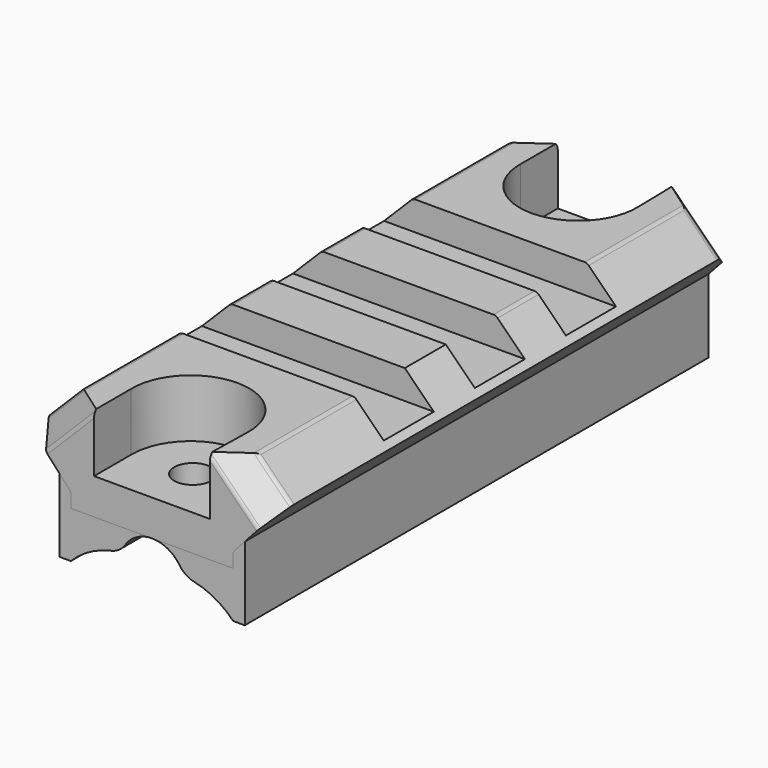
from build123d import *

# Parameters (mm, degrees)
F1_DEPTH  = 25
F2_W      = 28
F2_H      = 5.4
F2_W_2    = 13.9033808853
F2_W_3    = 14.6222274978
F3_DEPTH  = 2.5
F4_SIZE   = 2
F5_R      = 0.5
F8_DEPTH  = 5
F9_R      = 1.6
F10_DEPTH = 3.101
F12_DEPTH = 50
F14_R     = 2
F15_R     = 2
F17_R     = 1.6
F18_DEPTH = 47.90054


# Not quite as in the source:
# - a feature names something its author has since deleted; it is built from what else it names


with BuildPart() as f1:
    # F0 (on Front) → F1 (new body, symmetric)
    with BuildSketch(Plane.XZ):
        Polygon((-7.5, -4.8), (7.5, -4.8), (7.5, -3), (10.5, 0.3), (7.5, 3.3), (-7.5, 3.3), (-10.5, 0.3), (-7.5, -3), align=None)
    extrude(amount=F1_DEPTH, both=True)

    # F2 (on face) → F3 (cut)
    with BuildSketch(Plane.XY.offset(3.3)):
        Rectangle(F2_W, F2_H)
        Polygon((-14.1051735731, 12.5189756917), (-14, 7.12), (14.1193151165, 7.12), (14.1193151165, 12.5189756917), (0, 12.5189756917), align=None)
        with Locations((-6.9516904427, -9.8195246701)):
            Rectangle(F2_W_2, F2_H)
        with Locations((7.3111137489, -9.8195246701)):
            Rectangle(F2_W_3, F2_H)
    extrude(amount=-F3_DEPTH, mode=Mode.SUBTRACT)

    # F4
    f4_edges = [f1.edges().sort_by_distance(p)[0] for p in [
        (9, 25, 1.8),
        (-9, 25, 1.8),
        (9, -25, 1.8),
        (-9, -25, 1.8),
    ]]
    chamfer(f4_edges, length=F4_SIZE)

    # F5
    f5_edges = [f1.edges().sort_by_distance(p)[0] for p in [
        (-7.5, 17.759488, 3.3),
        (-7.5, 4.91, 3.3),
        (-7.5, -4.909762, 3.3),
        (-7.5, -17.759762, 3.3),
        (7.5, -17.759762, 3.3),
        (7.5, 4.91, 3.3),
        (7.5, 17.759488, 3.3),
        (-6.912351, 25, 1.059221),
        (9, 23, 1.8),
        (-9, 23, 1.8),
        (6.912351, -25, 1.059221),
        (9, -23, 1.8),
        (-6.912351, -25, 1.059221),
        (-9, -23, 1.8),
        (-7.5, -25, -3.9),
        (7.5, -25, -3.9),
        (7.5, 25, -3.9),
        (-7.5, 25, -3.9),
    ]]
    fillet(f5_edges, radius=F5_R)

    # F7 (on face) → F8 (cut)
    with BuildSketch(Plane.XY.offset(3.3)):
        with BuildLine():
            Line((-5, -25), (0, -25))
            Line((0, -25), (5, -25))
            Line((5, -25), (5.0857864376, -21.0009200199))
            ThreePointArc((5.0857864376, -21.0009200199), (0.0433631596, -15.8486988611), (-5, -21))
            Line((-5, -21), (-5, -25))
        make_face()
        with BuildLine():
            ThreePointArc((-5, 21), (0.0433631596, 15.8486988611), (5.0857864376, 21.0009200199))
            Line((5.0857864376, 21.0009200199), (5, 25))
            Line((5, 25), (-5, 25))
            Line((-5, 25), (-5, 21))
        make_face()
    extrude(amount=-F8_DEPTH, mode=Mode.SUBTRACT)

    # F9 (on face) → F10 (cut, through all)
    with BuildSketch(Plane.XY.offset(-1.7)):
        with Locations((0, -20.6)):
            Circle(F9_R)
        with Locations((0, 20.6)):
            Circle(F9_R)
    extrude(amount=-F10_DEPTH, mode=Mode.SUBTRACT)


with BuildPart() as f12:
    # F11 (on face) → F12 (new body)
    with BuildSketch(Plane.XZ.offset(25)):
        with BuildLine():
            ThreePointArc((-2.6432063896, -6.753962487), (-1.6435106798, -5.3415235892), (0, -4.8))
            Line((0, -4.8), (-2.5, -4.8))
            Line((-2.5, -4.8), (-7, -4.8))
            Line((-7, -4.8), (-7, -3.55))
            Line((-7, -3.55), (-8, -2.45))
            Line((-8, -2.45), (-8, -8.8))
            Line((-8, -8.8), (-7, -8.8))
            ThreePointArc((-7, -8.8), (-5.0036087462, -7.3894220622), (-2.6432063896, -6.753962487))
        make_face()
    extrude(amount=-F12_DEPTH)

    # F14
    f14_edges = [f12.edges().sort_by_distance(p)[0] for p in [
        (-2.643206, 0, -6.753962),
    ]]
    fillet(f14_edges, radius=F14_R)


with BuildPart() as f12b:
    # F11 (on face) → F12, piece 2 (new body)
    with BuildSketch(Plane.XZ.offset(25)):
        with BuildLine():
            Line((2.5, -4.8), (0, -4.8))
            ThreePointArc((0, -4.8), (1.6849251685, -5.3483353555), (2.724415157, -6.7832935601))
            ThreePointArc((2.724415157, -6.7832935601), (5.048675757, -7.396318783), (7, -8.8))
            Line((7, -8.8), (8, -8.8))
            Line((8, -8.8), (8, -2.45))
            Line((8, -2.45), (7, -3.55))
            Line((7, -3.55), (7, -4.8))
            Line((7, -4.8), (2.5, -4.8))
        make_face()
    extrude(amount=-F12_DEPTH)

    # F15
    f15_edges = [f12b.edges().sort_by_distance(p)[0] for p in [
        (2.724415, 0, -6.783294),
    ]]
    fillet(f15_edges, radius=F15_R)


with BuildPart() as f18_tool:
    # F17 (on offset) → F18 (new body)
    with BuildSketch(Plane.XY.offset(25)):
        with Locations((0, 20.606639777)):
            Circle(F17_R)
        with Locations((0, -20.5995866995)):
            Circle(F17_R)
    extrude(amount=-F18_DEPTH)


with BuildPart() as f12_1:
    add(f12.part)

    # F18: cut by f18_tool
    add(f18_tool.part, mode=Mode.SUBTRACT)


with BuildPart() as f12b_1:
    add(f12b.part)

    # F18: cut by f18_tool
    add(f18_tool.part, mode=Mode.SUBTRACT)


solid = Compound([f1.part, f12_1.part, f12b_1.part])
